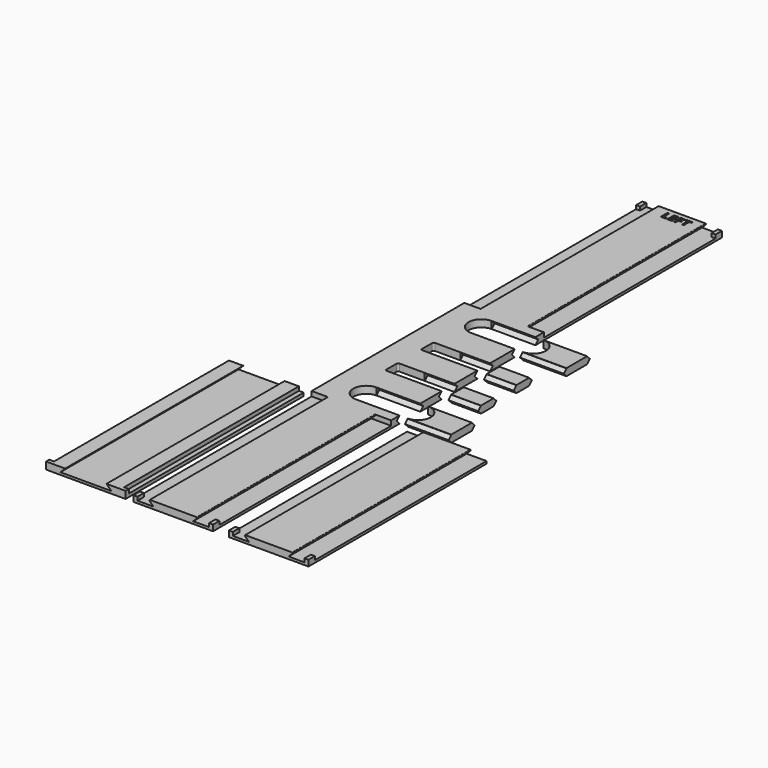
from build123d import *

# Parameters (mm, degrees)
F1_DEPTH      = 2.286
F0_W          = 25.4
F0_H          = 71.12
F0_W_2        = 9.525
F0_H_2        = 5.08
F0_H_3        = 5.0376876555
F3_DEPTH      = 71.12
F5_DEPTH      = 71.12
F6_W          = 1.27
F6_H          = 2.54
F7_DEPTH      = 1.143
F8_W          = 1.524
F8_H          = 69.85
F9_DEPTH      = 1.27
F11_DEPTH     = 13.97
F13_DEPTH     = 13.97
F16_DEPTH     = 9.525
F17_DEPTH     = 9.525
F18_TEXT_SIZE = 3.7573484911
F19_DEPTH     = 0.381


# Not quite as in the source:
# - Text() gives the source's letters only with a copy of the font that has no kerning and outlines rounded to 1/6400 em; it was checked with that copy


with BuildPart() as f1:
    # F0 (on Top) → F1 (new body)
    with BuildSketch(Plane.XY):
        with BuildLine():
            Line((-2.54, 131.2672), (-2.54, 205.74))
            Line((-2.54, 205.74), (-27.94, 205.74))
            Line((-27.94, 205.74), (-27.94, 2.54))
            Line((-27.94, 2.54), (-2.54, 2.54))
            Line((-2.54, 2.54), (-2.54, 77.0382))
            Line((-2.54, 77.0382), (-16.51, 77.0382))
            ThreePointArc((-16.51, 77.0382), (-20.6375, 81.1657), (-16.51, 85.2932))
            Line((-16.51, 85.2932), (-2.54, 85.2932))
            Line((-2.54, 85.2932), (-2.54, 93.8657))
            Line((-2.54, 93.8657), (-20.1295, 93.8657))
            ThreePointArc((-20.1295, 93.8657), (-20.4887102448, 94.0144897552), (-20.6375, 94.3737))
            Line((-20.6375, 94.3737), (-20.6375, 98.4377))
            ThreePointArc((-20.6375, 98.4377), (-20.4887102448, 98.7969102448), (-20.1295, 98.9457))
            Line((-20.1295, 98.9457), (-2.54, 98.9457))
            Line((-2.54, 98.9457), (-2.54, 108.0897))
            Line((-2.54, 108.0897), (-20.1295, 108.0897))
            ThreePointArc((-20.1295, 108.0897), (-20.4887102448, 108.2384897552), (-20.6375, 108.5977))
            Line((-20.6375, 108.5977), (-20.6375, 112.6617))
            ThreePointArc((-20.6375, 112.6617), (-20.4887102448, 113.0209102448), (-20.1295, 113.1697))
            Line((-20.1295, 113.1697), (-2.54, 113.1697))
            Line((-2.54, 113.1697), (-2.54, 123.0122))
            Line((-2.54, 123.0122), (-16.51, 123.0122))
            ThreePointArc((-16.51, 123.0122), (-20.6375, 127.1397), (-16.51, 131.2672))
            Line((-16.51, 131.2672), (-2.54, 131.2672))
        make_face()
    extrude(amount=F1_DEPTH)


with BuildPart() as f1b:
    # F0 (on Top) → F1, piece 2 (new body)
    with BuildSketch(Plane.XY):
        with Locations((-43.18, 38.1)):
            Rectangle(F0_W, F0_H)
    extrude(amount=F1_DEPTH)


with BuildPart() as f1c:
    # F0 (on Top) → F1, piece 3 (new body)
    with BuildSketch(Plane.XY):
        with Locations((15.24, 38.1)):
            Rectangle(F0_W, F0_H)
    extrude(amount=F1_DEPTH)


with BuildPart() as f1d:
    # F0 (on Top) → F1, piece 4 (new body)
    with BuildSketch(Plane.XY):
        with BuildLine():
            ThreePointArc((0, 85.2932), (4.1275, 81.1657), (0, 77.0382))
            Line((0, 77.0382), (13.97, 77.0382))
            Line((13.97, 77.0382), (13.97, 85.2932))
            Line((13.97, 85.2932), (0, 85.2932))
        make_face()
    extrude(amount=F1_DEPTH)

    # F12 (on face) → F13 (join)
    with BuildSketch(Plane.YZ.offset(13.97)):
        Polygon((77.0382, 0.0762), (77.0382, 2.2098), (75.9714, 1.143), align=None)
        Polygon((85.2932, 2.2098), (85.2932, 0.0762), (86.36, 1.143), align=None)
    extrude(amount=-F13_DEPTH)


with BuildPart() as f1e:
    # F0 (on Top) → F1, piece 5 (new body)
    with BuildSketch(Plane.XY):
        with BuildLine():
            ThreePointArc((0, 131.2672), (4.1275, 127.1397), (0, 123.0122))
            Line((0, 123.0122), (13.97, 123.0122))
            Line((13.97, 123.0122), (13.97, 131.2672))
            Line((13.97, 131.2672), (0, 131.2672))
        make_face()
    extrude(amount=F1_DEPTH)

    # F12 (on face) → F13, piece 2 (join)
    with BuildSketch(Plane.YZ.offset(13.97)):
        Polygon((123.0122, 0.0762), (123.0122, 2.2098), (121.9454, 1.143), align=None)
        Polygon((131.2672, 2.2098), (131.2672, 0.0762), (132.334, 1.143), align=None)
    extrude(amount=-F13_DEPTH)


with BuildPart() as f1f:
    # F0 (on Top) → F1, piece 6 (new body)
    with BuildSketch(Plane.XY):
        with Locations((5.1854069075, 110.6297)):
            Rectangle(F0_W_2, F0_H_2)
    extrude(amount=F1_DEPTH)

    # F14 (on face) → F17, piece 2 (join)
    with BuildSketch(Plane.YZ.offset(9.9479069075)):
        Polygon((108.0897, 0.0508), (108.0897, 2.2352), (106.9975, 1.143), align=None)
        Polygon((114.2619, 1.143), (113.1697, 2.2352), (113.1697, 0.0508), align=None)
    extrude(amount=-F17_DEPTH)


with BuildPart() as f1g:
    # F0 (on Top) → F1, piece 7 (new body)
    with BuildSketch(Plane.XY):
        with Locations((5.1854069075, 96.4268561723)):
            Rectangle(F0_W_2, F0_H_3)
    extrude(amount=F1_DEPTH)

    # F14 (on face) → F17 (join)
    with BuildSketch(Plane.YZ.offset(9.9479069075)):
        Polygon((93.9080123445, 0.0508), (93.9080123445, 2.2352), (92.8158123445, 1.143), align=None)
        Polygon((100.0379, 1.143), (98.9457, 2.2352), (98.9457, 0.0508), align=None)
    extrude(amount=-F17_DEPTH)


with BuildPart() as f3_tool:
    # F2 (on face) → F3 (new body)
    with BuildSketch(Plane.XZ.offset(-2.54)):
        with BuildLine():
            Line((-21.59, 0.762), (-22.8104764143, 1.9824764143))
            ThreePointArc((-22.8104764143, 1.9824764143), (-22.8490186095, 2.1762411143), (-22.6847528286, 2.286))
            Line((-22.6847528286, 2.286), (-27.94, 2.286))
            Line((-27.94, 2.286), (-27.94, 0.762))
            Line((-27.94, 0.762), (-21.59, 0.762))
        make_face()
        with BuildLine():
            Line((-7.6695235857, 1.9824764143), (-8.89, 0.762))
            Line((-8.89, 0.762), (-2.54, 0.762))
            Line((-2.54, 0.762), (-2.54, 2.286))
            Line((-2.54, 2.286), (-7.7952471714, 2.286))
            ThreePointArc((-7.7952471714, 2.286), (-7.6309813905, 2.1762411143), (-7.6695235857, 1.9824764143))
        make_face()
        Polygon((-36.576, 2.286), (-49.784, 2.286), (-51.308, 0.762), (-35.052, 0.762), align=None)
        with BuildLine():
            Line((7.7952471714, 2.286), (2.54, 2.286))
            Line((2.54, 2.286), (2.54, 0.762))
            Line((2.54, 0.762), (8.89, 0.762))
            Line((8.89, 0.762), (7.6695235857, 1.9824764143))
            ThreePointArc((7.6695235857, 1.9824764143), (7.6309813905, 2.1762411143), (7.7952471714, 2.286))
        make_face()
        with BuildLine():
            Line((21.59, 0.762), (27.94, 0.762))
            Line((27.94, 0.762), (27.94, 2.286))
            Line((27.94, 2.286), (22.6847528286, 2.286))
            ThreePointArc((22.6847528286, 2.286), (22.8490186095, 2.1762411143), (22.8104764143, 1.9824764143))
            Line((22.8104764143, 1.9824764143), (21.59, 0.762))
        make_face()
    extrude(amount=-F3_DEPTH)


with BuildPart() as f1_1:
    add(f1.part)

    # F3: cut by f3_tool
    add(f3_tool.part, mode=Mode.SUBTRACT)

    # F4 (on face) → F5 (cut)
    with BuildSketch(Plane(origin=(0, 205.74, 0), x_dir=(-1, 0, 0), z_dir=(0, 1, 0))):
        with BuildLine():
            Line((8.89, 0.762), (7.6695235857, 1.9824764143))
            ThreePointArc((7.6695235857, 1.9824764143), (7.6309813905, 2.1762411143), (7.7952471714, 2.286))
            Line((7.7952471714, 2.286), (2.54, 2.286))
            Line((2.54, 2.286), (2.54, 0.762))
            Line((2.54, 0.762), (8.89, 0.762))
        make_face()
        with BuildLine():
            Line((22.8104764143, 1.9824764143), (21.59, 0.762))
            Line((21.59, 0.762), (27.94, 0.762))
            Line((27.94, 0.762), (27.94, 2.286))
            Line((27.94, 2.286), (22.6847528286, 2.286))
            ThreePointArc((22.6847528286, 2.286), (22.8490186095, 2.1762411143), (22.8104764143, 1.9824764143))
        make_face()
    extrude(amount=-F5_DEPTH, mode=Mode.SUBTRACT)

    # F6 (on face) → F7, piece 2 (join)
    with BuildSketch(Plane.XY.offset(0.762)):
        with Locations((-3.175, 3.81)):
            Rectangle(F6_W, F6_H)
        with Locations((-27.305, 3.81)):
            Rectangle(F6_W, F6_H)
        with Locations((-27.305, 204.47)):
            Rectangle(F6_W, F6_H)
        with Locations((-3.175, 204.47)):
            Rectangle(F6_W, F6_H)
    extrude(amount=F7_DEPTH)

    # F10 (on face) → F11 (cut)
    with BuildSketch(Plane.YZ.offset(-2.54)):
        Polygon((86.4362, 1.143), (85.2932, 2.286), (85.2932, 0), align=None)
        Polygon((123.0122, 0), (123.0122, 2.286), (121.8692, 1.143), align=None)
        Polygon((132.4102, 1.143), (131.2672, 2.286), (131.2672, 0), align=None)
        Polygon((77.0382, 0), (77.0382, 2.286), (75.8952, 1.143), align=None)
    extrude(amount=-F11_DEPTH, mode=Mode.SUBTRACT)

    # F15 (on face) → F16 (cut)
    with BuildSketch(Plane.YZ.offset(-2.54)):
        Polygon((93.8657, 0), (93.8657, 2.286), (92.7227, 1.143), align=None)
        Polygon((100.0887, 1.143), (98.9457, 2.286), (98.9457, 0), align=None)
        Polygon((114.3127, 1.143), (113.1697, 2.286), (113.1697, 0), align=None)
        Polygon((108.0897, 0), (108.0897, 2.286), (106.9467, 1.143), align=None)
    extrude(amount=-F16_DEPTH, mode=Mode.SUBTRACT)

    # F18 (on face) → F19 (cut)
    with BuildSketch(Plane.XY.offset(2.286)):
        with Locations((-19.0785266459, 201.5499472618)):
            Text('LEFT', F18_TEXT_SIZE, font='Open Sans', font_style=FontStyle.BOLD, text_align=(TextAlign.LEFT, TextAlign.BOTTOM))
    extrude(amount=-F19_DEPTH, mode=Mode.SUBTRACT)


with BuildPart() as f1b_1:
    add(f1b.part)

    # F3: cut by f3_tool
    add(f3_tool.part, mode=Mode.SUBTRACT)

    # F8 (on face) → F9 (cut)
    with BuildSketch(Plane.XY.offset(2.286)):
        with Locations((-31.242, 38.735)):
            Rectangle(F8_W, F8_H)
        with Locations((-55.118, 38.735)):
            Rectangle(F8_W, F8_H)
    extrude(amount=-F9_DEPTH, mode=Mode.SUBTRACT)


with BuildPart() as f1c_1:
    add(f1c.part)

    # F3: cut by f3_tool
    add(f3_tool.part, mode=Mode.SUBTRACT)

    # F6 (on face) → F7 (join)
    with BuildSketch(Plane.XY.offset(0.762)):
        with Locations((27.305, 3.81)):
            Rectangle(F6_W, F6_H)
        with Locations((3.175, 3.81)):
            Rectangle(F6_W, F6_H)
    extrude(amount=F7_DEPTH)


solid = Compound([f1d.part, f1e.part, f1f.part, f1g.part, f1_1.part, f1b_1.part, f1c_1.part])
